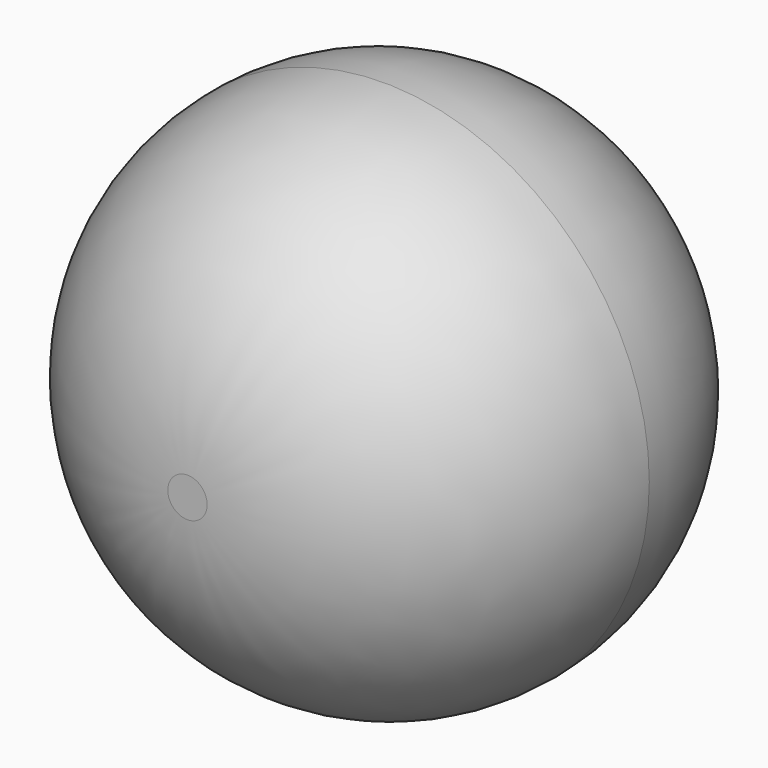
from build123d import *

# Parameters (mm, degrees)
F0_R     = 32.4022684909
F1_DEPTH = 60
F2_R     = 29.99999


# Not quite as in the source:
# - a fillet or chamfer is up to 0.001 mm smaller than in the source, because OpenCascade refuses the exact size


with BuildPart() as f1:
    # F0 (on Front) → F1 (new body)
    with BuildSketch(Plane.XZ):
        Circle(F0_R)
    extrude(amount=F1_DEPTH)

    # F2 (radius 30 in the source; OpenCascade refuses exactly that, so slightly less here)
    f2_edges = [f1.edges().sort_by_distance(p)[0] for p in [
        (-32.402268, -60, 0),
        (-32.402268, 0, 0),
    ]]
    fillet(f2_edges, radius=F2_R)


solid = f1.part
